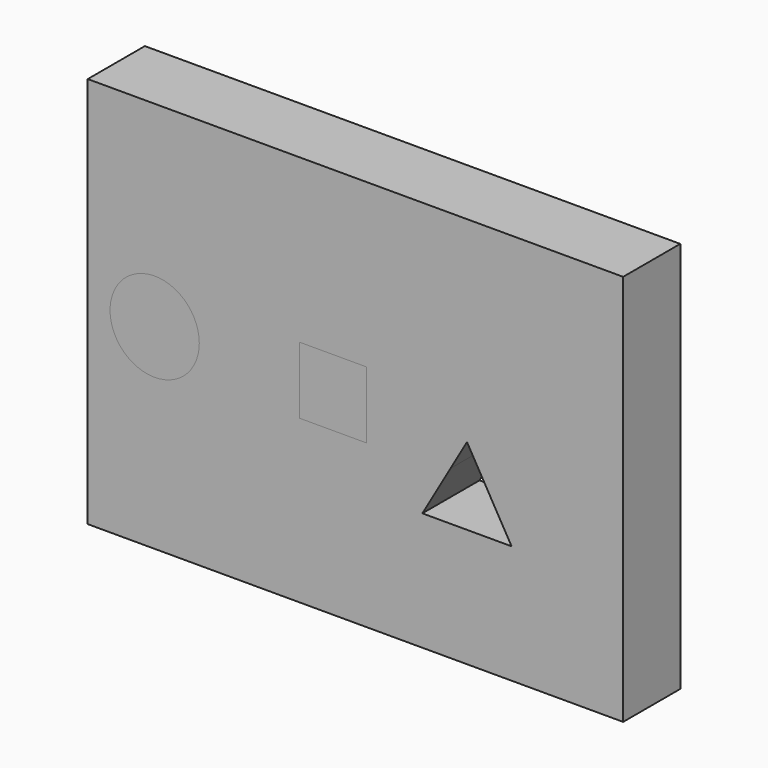
from build123d import *

# Parameters (mm, degrees)
F0_R     = 12.7
F1_DEPTH = 20.32
F2_DEPTH = 31.75
F3_DEPTH = 20.32


with BuildPart() as f1:
    # F0 (on Front) → F1 (new body)
    with BuildSketch(Plane.XZ):
        Polygon((50.8, -55.6751601398), (50.8, 0), (50.8, 55.8595135808), (-101.6, 55.8595135808), (-101.6, -55.6751601398), align=None)
        with Locations((-82.55, 0)):
            Circle(F0_R, mode=Mode.SUBTRACT)
        Polygon((-22.225, 9.525), (-22.225, 0), (-22.225, -9.525), (-41.275, -9.525), (-41.275, 0), (-41.275, 9.525), align=None, mode=Mode.SUBTRACT)
        Polygon((1.6667581252, -8.1116128713), (6.35, 0), (19.05, -21.9970452561), (-6.35, -21.9970452561), align=None, mode=Mode.SUBTRACT)
    extrude(amount=F1_DEPTH)


with BuildPart() as f2:
    # F0 (on Front) → F2 (new body)
    with BuildSketch(Plane.XZ):
        with Locations((-82.55, 0)):
            Circle(F0_R)
    extrude(amount=-F2_DEPTH)


with BuildPart() as f2b:
    # F0 (on Front) → F2, piece 2 (new body)
    with BuildSketch(Plane.XZ):
        Polygon((-22.225, -9.525), (-22.225, 0), (-31.75, 0), (-41.275, 0), (-41.275, -9.525), align=None)
        Polygon((-31.75, 0), (-22.225, 0), (-22.225, 9.525), (-41.275, 9.525), (-41.275, 0), align=None)
    extrude(amount=-F2_DEPTH)


with BuildPart() as f3:
    # F3 (new): a face of the model
    f3_faces = [f2.part.faces().sort_by_distance(p)[0] for p in [
        (-82.55, 0, 0),
    ]]
    extrude(f3_faces, amount=F3_DEPTH)


with BuildPart() as f3b:
    # F3#2 (new): a face of the model
    f3_2_faces = [f2b.part.faces().sort_by_distance(p)[0] for p in [
        (-31.75, 0, 0),
    ]]
    extrude(f3_2_faces, amount=F3_DEPTH)


solid = Compound([f1.part, f2.part, f2b.part, f3.part, f3b.part])
